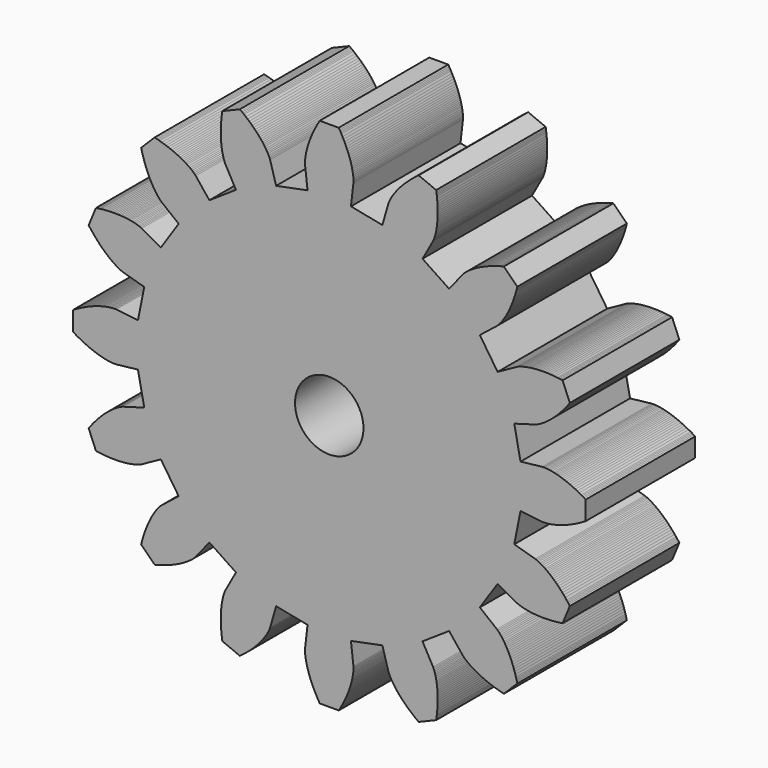
from build123d import *

# Parameters (mm, degrees)
F0_R     = 1.5
F1_DEPTH = 6


# Not quite as in the source:
# - ends of sketch curves that miss each other by under 0.0002 mm in the source are joined


with BuildPart() as f1:
    # F0 (on Front) → F1 (new body)
    with BuildSketch(Plane.XZ):
        with BuildLine():
            ThreePointArc((8.1098128622, -2.3285659726), (8.2466730878, -1.6403675501), (8.3835933696, -0.9521810736))
            Line((8.3835933696, -0.9521810736), (9.336897, -1.060451))
            Line((9.336897, -1.060451), (9.388357, -1.06268))
            Line((9.388357, -1.06268), (9.44023, -1.061917))
            Line((9.44023, -1.061917), (9.494537, -1.059018))
            Line((9.494537, -1.059018), (9.560114, -1.053224))
            Line((9.560114, -1.053224), (9.616606, -1.046504))
            Line((9.616606, -1.046504), (9.679275, -1.03738))
            Line((9.679275, -1.03738), (9.748033, -1.025526))
            Line((9.748033, -1.025526), (9.822771, -1.010618))
            Line((9.822771, -1.010618), (9.875862, -0.998824))
            Line((9.875862, -0.998824), (9.931523, -0.985435))
            Line((9.931523, -0.985435), (9.989713, -0.97036))
            Line((9.989713, -0.97036), (10.05039, -0.953506))
            Line((10.05039, -0.953506), (10.113507, -0.934781))
            Line((10.113507, -0.934781), (10.179017, -0.914096))
            Line((10.179017, -0.914096), (10.24687, -0.891361))
            Line((10.24687, -0.891361), (10.317014, -0.866489))
            Line((10.317014, -0.866489), (10.389394, -0.839394))
            Line((10.389394, -0.839394), (10.463954, -0.809989))
            Line((10.463954, -0.809989), (10.540633, -0.778191))
            Line((10.540633, -0.778191), (10.61937, -0.743918))
            Line((10.61937, -0.743918), (10.7001, -0.707087))
            Line((10.7001, -0.707087), (10.78276, -0.667621))
            Line((10.78276, -0.667621), (10.867278, -0.625439))
            Line((10.867278, -0.625439), (10.953587, -0.580466))
            Line((10.953587, -0.580466), (11.041613, -0.532627))
            Line((11.041613, -0.532627), (11.086246, -0.50761))
            Line((11.086246, -0.50761), (11.13128, -0.481849))
            Line((11.13128, -0.481849), (11.176706, -0.455335))
            Line((11.176706, -0.455335), (11.242303, -0.416041))
            Line((11.242303, -0.416041), (11.242301, 0.416042))
            Line((11.242301, 0.416042), (11.176705, 0.455336))
            Line((11.176705, 0.455336), (11.13128, 0.48185))
            Line((11.13128, 0.48185), (11.086245, 0.507611))
            Line((11.086245, 0.507611), (11.041612, 0.532628))
            Line((11.041612, 0.532628), (10.953587, 0.580467))
            Line((10.953587, 0.580467), (10.867277, 0.62544))
            Line((10.867277, 0.62544), (10.782758, 0.667622))
            Line((10.782758, 0.667622), (10.7001, 0.707089))
            Line((10.7001, 0.707089), (10.619369, 0.743919))
            Line((10.619369, 0.743919), (10.540632, 0.778193))
            Line((10.540632, 0.778193), (10.463953, 0.809991))
            Line((10.463953, 0.809991), (10.389394, 0.839395))
            Line((10.389394, 0.839395), (10.317014, 0.866491))
            Line((10.317014, 0.866491), (10.24687, 0.891362))
            Line((10.24687, 0.891362), (10.179016, 0.914097))
            Line((10.179016, 0.914097), (10.113507, 0.934782))
            Line((10.113507, 0.934782), (10.05039, 0.953507))
            Line((10.05039, 0.953507), (9.989712, 0.970362))
            Line((9.989712, 0.970362), (9.931522, 0.985437))
            Line((9.931522, 0.985437), (9.875862, 0.998825))
            Line((9.875862, 0.998825), (9.82277, 1.010619))
            Line((9.82277, 1.010619), (9.748032, 1.025527))
            Line((9.748032, 1.025527), (9.679275, 1.037381))
            Line((9.679275, 1.037381), (9.616605, 1.046505))
            Line((9.616605, 1.046505), (9.560113, 1.053226))
            Line((9.560113, 1.053226), (9.494536, 1.05902))
            Line((9.494536, 1.05902), (9.440229, 1.061919))
            Line((9.440229, 1.061919), (9.388357, 1.062681))
            Line((9.388357, 1.062681), (9.336897, 1.060452))
            Line((9.336897, 1.060452), (8.383598, 0.952181))
            ThreePointArc((8.383598, 0.952181), (8.2466779536, 1.640366924), (8.1098182701, 2.3285648549))
            Line((8.1098182701, 2.3285648549), (9.031984, 2.593346))
            Line((9.031984, 2.593346), (9.08038, 2.61098))
            Line((9.08038, 2.61098), (9.128012, 2.631536))
            Line((9.128012, 2.631536), (9.177077, 2.654996))
            Line((9.177077, 2.654996), (9.235444, 2.685445))
            Line((9.235444, 2.685445), (9.285064, 2.713272))
            Line((9.285064, 2.713272), (9.339471, 2.745684))
            Line((9.339471, 2.745684), (9.398459, 2.782947))
            Line((9.398459, 2.782947), (9.461803, 2.825322))
            Line((9.461803, 2.825322), (9.50634, 2.856535))
            Line((9.50634, 2.856535), (9.55264, 2.890205))
            Line((9.55264, 2.890205), (9.600631, 2.926401))
            Line((9.600631, 2.926401), (9.65024, 2.965193))
            Line((9.65024, 2.965193), (9.701386, 3.006646))
            Line((9.701386, 3.006646), (9.753994, 3.050826))
            Line((9.753994, 3.050826), (9.807982, 3.097797))
            Line((9.807982, 3.097797), (9.863268, 3.147618))
            Line((9.863268, 3.147618), (9.91977, 3.20035))
            Line((9.91977, 3.20035), (9.977402, 3.256049))
            Line((9.977402, 3.256049), (10.036075, 3.31477))
            Line((10.036075, 3.31477), (10.095703, 3.376566))
            Line((10.095703, 3.376566), (10.156193, 3.441487))
            Line((10.156193, 3.441487), (10.217458, 3.509582))
            Line((10.217458, 3.509582), (10.279401, 3.580897))
            Line((10.279401, 3.580897), (10.341929, 3.655475))
            Line((10.341929, 3.655475), (10.404946, 3.733358))
            Line((10.404946, 3.733358), (10.436609, 3.773552))
            Line((10.436609, 3.773552), (10.468356, 3.814586))
            Line((10.468356, 3.814586), (10.500178, 3.856465))
            Line((10.500178, 3.856465), (10.545745, 3.91787))
            Line((10.545745, 3.91787), (10.227319, 4.686615))
            Line((10.227319, 4.686615), (10.151679, 4.697815))
            Line((10.151679, 4.697815), (10.099564, 4.704927))
            Line((10.099564, 4.704927), (10.0481, 4.711493))
            Line((10.0481, 4.711493), (9.997291, 4.717525))
            Line((9.997291, 4.717525), (9.897658, 4.728037))
            Line((9.897658, 4.728037), (9.800709, 4.736558))
            Line((9.800709, 4.736558), (9.706481, 4.743185))
            Line((9.706481, 4.743185), (9.615012, 4.748015))
            Line((9.615012, 4.748015), (9.526332, 4.751148))
            Line((9.526332, 4.751148), (9.440472, 4.752681))
            Line((9.440472, 4.752681), (9.357462, 4.752715))
            Line((9.357462, 4.752715), (9.277326, 4.751348))
            Line((9.277326, 4.751348), (9.200086, 4.748683))
            Line((9.200086, 4.748683), (9.125763, 4.744818))
            Line((9.125763, 4.744818), (9.054374, 4.739856))
            Line((9.054374, 4.739856), (8.985936, 4.733897))
            Line((8.985936, 4.733897), (8.920458, 4.727043))
            Line((8.920458, 4.727043), (8.857949, 4.719394))
            Line((8.857949, 4.719394), (8.798419, 4.711053))
            Line((8.798419, 4.711053), (8.741873, 4.702122))
            Line((8.741873, 4.702122), (8.688308, 4.692701))
            Line((8.688308, 4.692701), (8.613554, 4.677873))
            Line((8.613554, 4.677873), (8.545495, 4.662513))
            Line((8.545495, 4.662513), (8.484104, 4.646959))
            Line((8.484104, 4.646959), (8.42934, 4.63155))
            Line((8.42934, 4.63155), (8.366538, 4.611807))
            Line((8.366538, 4.611807), (8.315254, 4.593703))
            Line((8.315254, 4.593703), (8.26704, 4.574557))
            Line((8.26704, 4.574557), (8.22035, 4.552805))
            Line((8.22035, 4.552805), (7.38105, 4.087963))
            ThreePointArc((7.38105, 4.087963), (6.9911949356, 4.6713679184), (6.6013908032, 5.2548068685))
            Line((6.6013908032, 5.2548068685), (7.352035, 5.852329))
            Line((7.352035, 5.852329), (7.389998, 5.887142))
            Line((7.389998, 5.887142), (7.426139, 5.92436))
            Line((7.426139, 5.92436), (7.46249, 5.964811))
            Line((7.46249, 5.964811), (7.504763, 6.015278))
            Line((7.504763, 6.015278), (7.539957, 6.059976))
            Line((7.539957, 6.059976), (7.577818, 6.110741))
            Line((7.577818, 6.110741), (7.618056, 6.167742))
            Line((7.618056, 6.167742), (7.660361, 6.231132))
            Line((7.660361, 6.231132), (7.689563, 6.277012))
            Line((7.689563, 6.277012), (7.719454, 6.325838))
            Line((7.719454, 6.325838), (7.749941, 6.377644))
            Line((7.749941, 6.377644), (7.780928, 6.432466))
            Line((7.780928, 6.432466), (7.812318, 6.490337))
            Line((7.812318, 6.490337), (7.844014, 6.551287))
            Line((7.844014, 6.551287), (7.875918, 6.615342))
            Line((7.875918, 6.615342), (7.907931, 6.682528))
            Line((7.907931, 6.682528), (7.939951, 6.752868))
            Line((7.939951, 6.752868), (7.971881, 6.826382))
            Line((7.971881, 6.826382), (8.003616, 6.903087))
            Line((8.003616, 6.903087), (8.035057, 6.982997))
            Line((8.035057, 6.982997), (8.066099, 7.066125))
            Line((8.066099, 7.066125), (8.096641, 7.152482))
            Line((8.096641, 7.152482), (8.126577, 7.242073))
            Line((8.126577, 7.242073), (8.155806, 7.334903))
            Line((8.155806, 7.334903), (8.184222, 7.430973))
            Line((8.184222, 7.430973), (8.198093, 7.480224))
            Line((8.198093, 7.480224), (8.211721, 7.530283))
            Line((8.211721, 7.530283), (8.225094, 7.581152))
            Line((8.225094, 7.581152), (8.243693, 7.65532))
            Line((8.243693, 7.65532), (7.65532, 8.243692))
            Line((7.65532, 8.243692), (7.581153, 8.225093))
            Line((7.581153, 8.225093), (7.530283, 8.211721))
            Line((7.530283, 8.211721), (7.480223, 8.198092))
            Line((7.480223, 8.198092), (7.430973, 8.184222))
            Line((7.430973, 8.184222), (7.334902, 8.155806))
            Line((7.334902, 8.155806), (7.242072, 8.126577))
            Line((7.242072, 8.126577), (7.152481, 8.096639))
            Line((7.152481, 8.096639), (7.066126, 8.066099))
            Line((7.066126, 8.066099), (6.982996, 8.035057))
            Line((6.982996, 8.035057), (6.903087, 8.003616))
            Line((6.903087, 8.003616), (6.826382, 7.97188))
            Line((6.826382, 7.97188), (6.752868, 7.939951))
            Line((6.752868, 7.939951), (6.682529, 7.90793))
            Line((6.682529, 7.90793), (6.615342, 7.875918))
            Line((6.615342, 7.875918), (6.551286, 7.844014))
            Line((6.551286, 7.844014), (6.490338, 7.812318))
            Line((6.490338, 7.812318), (6.432467, 7.780927))
            Line((6.432467, 7.780927), (6.377643, 7.749941))
            Line((6.377643, 7.749941), (6.325837, 7.719454))
            Line((6.325837, 7.719454), (6.277012, 7.689563))
            Line((6.277012, 7.689563), (6.231131, 7.660361))
            Line((6.231131, 7.660361), (6.167742, 7.618055))
            Line((6.167742, 7.618055), (6.110741, 7.577819))
            Line((6.110741, 7.577819), (6.059976, 7.539955))
            Line((6.059976, 7.539955), (6.015278, 7.504762))
            Line((6.015278, 7.504762), (5.96481, 7.462488))
            Line((5.96481, 7.462488), (5.92436, 7.426137))
            Line((5.92436, 7.426137), (5.887141, 7.389998))
            Line((5.887141, 7.389998), (5.85233, 7.352035))
            Line((5.85233, 7.352035), (5.254806, 6.601391))
            ThreePointArc((5.254806, 6.601391), (4.6713678902, 6.9911948934), (4.0879640006, 7.3810500008))
            Line((4.0879640006, 7.3810500008), (4.552805, 8.220348))
            Line((4.552805, 8.220348), (4.574556, 8.267039))
            Line((4.574556, 8.267039), (4.593703, 8.315255))
            Line((4.593703, 8.315255), (4.611807, 8.366537))
            Line((4.611807, 8.366537), (4.631549, 8.429341))
            Line((4.631549, 8.429341), (4.646959, 8.484103))
            Line((4.646959, 8.484103), (4.662513, 8.545494))
            Line((4.662513, 8.545494), (4.677873, 8.613554))
            Line((4.677873, 8.613554), (4.6927, 8.688308))
            Line((4.6927, 8.688308), (4.702121, 8.741871))
            Line((4.702121, 8.741871), (4.711053, 8.798419))
            Line((4.711053, 8.798419), (4.719393, 8.857949))
            Line((4.719393, 8.857949), (4.727042, 8.920456))
            Line((4.727042, 8.920456), (4.733896, 8.985934))
            Line((4.733896, 8.985934), (4.739855, 9.054374))
            Line((4.739855, 9.054374), (4.744818, 9.125763))
            Line((4.744818, 9.125763), (4.748682, 9.200085))
            Line((4.748682, 9.200085), (4.751347, 9.277325))
            Line((4.751347, 9.277325), (4.752714, 9.357462))
            Line((4.752714, 9.357462), (4.75268, 9.440471))
            Line((4.75268, 9.440471), (4.751147, 9.526331))
            Line((4.751147, 9.526331), (4.748014, 9.61501))
            Line((4.748014, 9.61501), (4.743184, 9.706481))
            Line((4.743184, 9.706481), (4.736557, 9.800708))
            Line((4.736557, 9.800708), (4.728037, 9.897657))
            Line((4.728037, 9.897657), (4.717525, 9.99729))
            Line((4.717525, 9.99729), (4.711492, 10.048099))
            Line((4.711492, 10.048099), (4.704926, 10.099564))
            Line((4.704926, 10.099564), (4.697815, 10.151679))
            Line((4.697815, 10.151679), (4.686615, 10.227319))
            Line((4.686615, 10.227319), (3.917869, 10.545742))
            Line((3.917869, 10.545742), (3.856464, 10.500177))
            Line((3.856464, 10.500177), (3.814585, 10.468356))
            Line((3.814585, 10.468356), (3.773551, 10.436607))
            Line((3.773551, 10.436607), (3.733358, 10.404945))
            Line((3.733358, 10.404945), (3.655474, 10.341927))
            Line((3.655474, 10.341927), (3.580896, 10.279398))
            Line((3.580896, 10.279398), (3.509581, 10.217455))
            Line((3.509581, 10.217455), (3.441486, 10.156192))
            Line((3.441486, 10.156192), (3.376565, 10.095701))
            Line((3.376565, 10.095701), (3.314769, 10.036073))
            Line((3.314769, 10.036073), (3.256047, 9.9774))
            Line((3.256047, 9.9774), (3.200349, 9.919769))
            Line((3.200349, 9.919769), (3.147617, 9.863268))
            Line((3.147617, 9.863268), (3.097796, 9.807982))
            Line((3.097796, 9.807982), (3.050826, 9.753992))
            Line((3.050826, 9.753992), (3.006645, 9.701385))
            Line((3.006645, 9.701385), (2.965192, 9.650238))
            Line((2.965192, 9.650238), (2.9264, 9.60063))
            Line((2.9264, 9.60063), (2.890204, 9.552638))
            Line((2.890204, 9.552638), (2.856535, 9.506338))
            Line((2.856535, 9.506338), (2.825321, 9.461801))
            Line((2.825321, 9.461801), (2.782947, 9.398458))
            Line((2.782947, 9.398458), (2.745683, 9.339471))
            Line((2.745683, 9.339471), (2.713271, 9.285062))
            Line((2.713271, 9.285062), (2.685444, 9.235443))
            Line((2.685444, 9.235443), (2.654995, 9.177075))
            Line((2.654995, 9.177075), (2.631534, 9.128011))
            Line((2.631534, 9.128011), (2.61098, 9.080379))
            Line((2.61098, 9.080379), (2.593345, 9.031984))
            Line((2.593345, 9.031984), (2.328564, 8.109817))
            ThreePointArc((2.328564, 8.109817), (1.6403660669, 8.2466771725), (0.9521800641, 8.3835973224))
            Line((0.9521800641, 8.3835973224), (1.060452, 9.336894))
            Line((1.060452, 9.336894), (1.06268, 9.388354))
            Line((1.06268, 9.388354), (1.061918, 9.440227))
            Line((1.061918, 9.440227), (1.059019, 9.494534))
            Line((1.059019, 9.494534), (1.053225, 9.560111))
            Line((1.053225, 9.560111), (1.046504, 9.616603))
            Line((1.046504, 9.616603), (1.03738, 9.679273))
            Line((1.03738, 9.679273), (1.025527, 9.74803))
            Line((1.025527, 9.74803), (1.010618, 9.822768))
            Line((1.010618, 9.822768), (0.998824, 9.875859))
            Line((0.998824, 9.875859), (0.985436, 9.931521))
            Line((0.985436, 9.931521), (0.970361, 9.98971))
            Line((0.970361, 9.98971), (0.953506, 10.050387))
            Line((0.953506, 10.050387), (0.934781, 10.113504))
            Line((0.934781, 10.113504), (0.914096, 10.179013))
            Line((0.914096, 10.179013), (0.891362, 10.246867))
            Line((0.891362, 10.246867), (0.86649, 10.317011))
            Line((0.86649, 10.317011), (0.839394, 10.389391))
            Line((0.839394, 10.389391), (0.80999, 10.463951))
            Line((0.80999, 10.463951), (0.778192, 10.540629))
            Line((0.778192, 10.540629), (0.743918, 10.619366))
            Line((0.743918, 10.619366), (0.707088, 10.700097))
            Line((0.707088, 10.700097), (0.667621, 10.782756))
            Line((0.667621, 10.782756), (0.62544, 10.867275))
            Line((0.62544, 10.867275), (0.580467, 10.953583))
            Line((0.580467, 10.953583), (0.532628, 11.041609))
            Line((0.532628, 11.041609), (0.50761, 11.086242))
            Line((0.50761, 11.086242), (0.481849, 11.131276))
            Line((0.481849, 11.131276), (0.455335, 11.176703))
            Line((0.455335, 11.176703), (0.416042, 11.242299))
            Line((0.416042, 11.242299), (-0.416042, 11.242299))
            Line((-0.416042, 11.242299), (-0.455335, 11.176703))
            Line((-0.455335, 11.176703), (-0.481849, 11.131277))
            Line((-0.481849, 11.131277), (-0.50761, 11.086242))
            Line((-0.50761, 11.086242), (-0.532628, 11.041609))
            Line((-0.532628, 11.041609), (-0.580466, 10.953584))
            Line((-0.580466, 10.953584), (-0.62544, 10.867275))
            Line((-0.62544, 10.867275), (-0.667621, 10.782756))
            Line((-0.667621, 10.782756), (-0.707088, 10.700097))
            Line((-0.707088, 10.700097), (-0.743918, 10.619366))
            Line((-0.743918, 10.619366), (-0.778192, 10.540629))
            Line((-0.778192, 10.540629), (-0.80999, 10.46395))
            Line((-0.80999, 10.46395), (-0.839395, 10.389392))
            Line((-0.839395, 10.389392), (-0.86649, 10.317011))
            Line((-0.86649, 10.317011), (-0.891362, 10.246868))
            Line((-0.891362, 10.246868), (-0.914096, 10.179013))
            Line((-0.914096, 10.179013), (-0.934781, 10.113504))
            Line((-0.934781, 10.113504), (-0.953506, 10.050388))
            Line((-0.953506, 10.050388), (-0.970361, 9.98971))
            Line((-0.970361, 9.98971), (-0.985436, 9.93152))
            Line((-0.985436, 9.93152), (-0.998824, 9.87586))
            Line((-0.998824, 9.87586), (-1.010618, 9.822768))
            Line((-1.010618, 9.822768), (-1.025527, 9.74803))
            Line((-1.025527, 9.74803), (-1.037381, 9.679273))
            Line((-1.037381, 9.679273), (-1.046504, 9.616603))
            Line((-1.046504, 9.616603), (-1.053225, 9.560111))
            Line((-1.053225, 9.560111), (-1.059019, 9.494534))
            Line((-1.059019, 9.494534), (-1.061918, 9.440227))
            Line((-1.061918, 9.440227), (-1.06268, 9.388355))
            Line((-1.06268, 9.388355), (-1.060452, 9.336895))
            Line((-1.060452, 9.336895), (-0.95218, 8.383596))
            ThreePointArc((-0.95218, 8.383596), (-1.6403666784, 8.2466772329), (-2.3285650902, 8.1098174538))
            Line((-2.3285650902, 8.1098174538), (-2.593346, 9.031983))
            Line((-2.593346, 9.031983), (-2.61098, 9.080378))
            Line((-2.61098, 9.080378), (-2.631535, 9.128011))
            Line((-2.631535, 9.128011), (-2.654996, 9.177075))
            Line((-2.654996, 9.177075), (-2.685444, 9.235442))
            Line((-2.685444, 9.235442), (-2.713272, 9.285061))
            Line((-2.713272, 9.285061), (-2.745683, 9.33947))
            Line((-2.745683, 9.33947), (-2.782947, 9.398457))
            Line((-2.782947, 9.398457), (-2.825322, 9.461801))
            Line((-2.825322, 9.461801), (-2.856535, 9.506337))
            Line((-2.856535, 9.506337), (-2.890205, 9.552638))
            Line((-2.890205, 9.552638), (-2.926401, 9.600629))
            Line((-2.926401, 9.600629), (-2.965192, 9.650237))
            Line((-2.965192, 9.650237), (-3.006645, 9.701384))
            Line((-3.006645, 9.701384), (-3.050826, 9.753992))
            Line((-3.050826, 9.753992), (-3.097796, 9.80798))
            Line((-3.097796, 9.80798), (-3.147618, 9.863266))
            Line((-3.147618, 9.863266), (-3.20035, 9.919768))
            Line((-3.20035, 9.919768), (-3.256049, 9.9774))
            Line((-3.256049, 9.9774), (-3.314769, 10.036073))
            Line((-3.314769, 10.036073), (-3.376566, 10.0957))
            Line((-3.376566, 10.0957), (-3.441487, 10.156191))
            Line((-3.441487, 10.156191), (-3.509582, 10.217456))
            Line((-3.509582, 10.217456), (-3.580896, 10.279398))
            Line((-3.580896, 10.279398), (-3.655475, 10.341926))
            Line((-3.655475, 10.341926), (-3.733358, 10.404944))
            Line((-3.733358, 10.404944), (-3.773552, 10.436606))
            Line((-3.773552, 10.436606), (-3.814586, 10.468354))
            Line((-3.814586, 10.468354), (-3.856465, 10.500176))
            Line((-3.856465, 10.500176), (-3.91787, 10.545743))
            Line((-3.91787, 10.545743), (-4.686615, 10.227317))
            Line((-4.686615, 10.227317), (-4.697815, 10.151677))
            Line((-4.697815, 10.151677), (-4.704926, 10.099563))
            Line((-4.704926, 10.099563), (-4.711492, 10.048098))
            Line((-4.711492, 10.048098), (-4.717525, 9.997289))
            Line((-4.717525, 9.997289), (-4.728037, 9.897656))
            Line((-4.728037, 9.897656), (-4.736557, 9.800707))
            Line((-4.736557, 9.800707), (-4.743185, 9.706479))
            Line((-4.743185, 9.706479), (-4.748015, 9.61501))
            Line((-4.748015, 9.61501), (-4.751147, 9.526329))
            Line((-4.751147, 9.526329), (-4.75268, 9.44047))
            Line((-4.75268, 9.44047), (-4.752715, 9.357459))
            Line((-4.752715, 9.357459), (-4.751348, 9.277324))
            Line((-4.751348, 9.277324), (-4.748682, 9.200084))
            Line((-4.748682, 9.200084), (-4.744818, 9.125762))
            Line((-4.744818, 9.125762), (-4.739855, 9.054372))
            Line((-4.739855, 9.054372), (-4.733896, 8.985934))
            Line((-4.733896, 8.985934), (-4.727042, 8.920456))
            Line((-4.727042, 8.920456), (-4.719393, 8.857947))
            Line((-4.719393, 8.857947), (-4.711053, 8.798417))
            Line((-4.711053, 8.798417), (-4.702122, 8.741871))
            Line((-4.702122, 8.741871), (-4.6927, 8.688307))
            Line((-4.6927, 8.688307), (-4.677873, 8.613552))
            Line((-4.677873, 8.613552), (-4.662513, 8.545494))
            Line((-4.662513, 8.545494), (-4.646959, 8.484103))
            Line((-4.646959, 8.484103), (-4.631549, 8.429338))
            Line((-4.631549, 8.429338), (-4.611807, 8.366536))
            Line((-4.611807, 8.366536), (-4.593703, 8.315254))
            Line((-4.593703, 8.315254), (-4.574556, 8.267038))
            Line((-4.574556, 8.267038), (-4.552805, 8.220348))
            Line((-4.552805, 8.220348), (-4.087963, 7.38105))
            ThreePointArc((-4.087963, 7.38105), (-4.671367156, 6.9911945428), (-5.254805702, 6.6013905539))
            Line((-5.254805702, 6.6013905539), (-5.85233, 7.352033))
            Line((-5.85233, 7.352033), (-5.887142, 7.389997))
            Line((-5.887142, 7.389997), (-5.924361, 7.426137))
            Line((-5.924361, 7.426137), (-5.964812, 7.462489))
            Line((-5.964812, 7.462489), (-6.015279, 7.504761))
            Line((-6.015279, 7.504761), (-6.059977, 7.539955))
            Line((-6.059977, 7.539955), (-6.110742, 7.577818))
            Line((-6.110742, 7.577818), (-6.167742, 7.618054))
            Line((-6.167742, 7.618054), (-6.231132, 7.66036))
            Line((-6.231132, 7.66036), (-6.277013, 7.689562))
            Line((-6.277013, 7.689562), (-6.325838, 7.719454))
            Line((-6.325838, 7.719454), (-6.377645, 7.749941))
            Line((-6.377645, 7.749941), (-6.432468, 7.780927))
            Line((-6.432468, 7.780927), (-6.490339, 7.812317))
            Line((-6.490339, 7.812317), (-6.551288, 7.844013))
            Line((-6.551288, 7.844013), (-6.615343, 7.875917))
            Line((-6.615343, 7.875917), (-6.68253, 7.907929))
            Line((-6.68253, 7.907929), (-6.75287, 7.939951))
            Line((-6.75287, 7.939951), (-6.826384, 7.971881))
            Line((-6.826384, 7.971881), (-6.903087, 8.003616))
            Line((-6.903087, 8.003616), (-6.982998, 8.035056))
            Line((-6.982998, 8.035056), (-7.066126, 8.066097))
            Line((-7.066126, 8.066097), (-7.152483, 8.09664))
            Line((-7.152483, 8.09664), (-7.242073, 8.126576))
            Line((-7.242073, 8.126576), (-7.334904, 8.155805))
            Line((-7.334904, 8.155805), (-7.430974, 8.184222))
            Line((-7.430974, 8.184222), (-7.480225, 8.198092))
            Line((-7.480225, 8.198092), (-7.530285, 8.21172))
            Line((-7.530285, 8.21172), (-7.581154, 8.225093))
            Line((-7.581154, 8.225093), (-7.655322, 8.243692))
            Line((-7.655322, 8.243692), (-8.243693, 7.655319))
            Line((-8.243693, 7.655319), (-8.225094, 7.581152))
            Line((-8.225094, 7.581152), (-8.211722, 7.530283))
            Line((-8.211722, 7.530283), (-8.198093, 7.480222))
            Line((-8.198093, 7.480222), (-8.184224, 7.430972))
            Line((-8.184224, 7.430972), (-8.155807, 7.334902))
            Line((-8.155807, 7.334902), (-8.126578, 7.242071))
            Line((-8.126578, 7.242071), (-8.09664, 7.15248))
            Line((-8.09664, 7.15248), (-8.0661, 7.066124))
            Line((-8.0661, 7.066124), (-8.035057, 6.982996))
            Line((-8.035057, 6.982996), (-8.003617, 6.903085))
            Line((-8.003617, 6.903085), (-7.971881, 6.826381))
            Line((-7.971881, 6.826381), (-7.939953, 6.752868))
            Line((-7.939953, 6.752868), (-7.907932, 6.682527))
            Line((-7.907932, 6.682527), (-7.875919, 6.615342))
            Line((-7.875919, 6.615342), (-7.844015, 6.551286))
            Line((-7.844015, 6.551286), (-7.812319, 6.490337))
            Line((-7.812319, 6.490337), (-7.780929, 6.432466))
            Line((-7.780929, 6.432466), (-7.749943, 6.377643))
            Line((-7.749943, 6.377643), (-7.719455, 6.325837))
            Line((-7.719455, 6.325837), (-7.689564, 6.277012))
            Line((-7.689564, 6.277012), (-7.660362, 6.23113))
            Line((-7.660362, 6.23113), (-7.618056, 6.167741))
            Line((-7.618056, 6.167741), (-7.57782, 6.110741))
            Line((-7.57782, 6.110741), (-7.539957, 6.059975))
            Line((-7.539957, 6.059975), (-7.504763, 6.015277))
            Line((-7.504763, 6.015277), (-7.46249, 5.96481))
            Line((-7.46249, 5.96481), (-7.426139, 5.924359))
            Line((-7.426139, 5.924359), (-7.389998, 5.887141))
            Line((-7.389998, 5.887141), (-7.352036, 5.852329))
            Line((-7.352036, 5.852329), (-6.601392, 5.254806))
            ThreePointArc((-6.601392, 5.254806), (-6.9911965642, 4.6713675043), (-7.381052057, 4.0879630381))
            Line((-7.381052057, 4.0879630381), (-8.22035, 4.552805))
            Line((-8.22035, 4.552805), (-8.267042, 4.574556))
            Line((-8.267042, 4.574556), (-8.315257, 4.593703))
            Line((-8.315257, 4.593703), (-8.366539, 4.611808))
            Line((-8.366539, 4.611808), (-8.429343, 4.631549))
            Line((-8.429343, 4.631549), (-8.484105, 4.646959))
            Line((-8.484105, 4.646959), (-8.545496, 4.662512))
            Line((-8.545496, 4.662512), (-8.613556, 4.677873))
            Line((-8.613556, 4.677873), (-8.68831, 4.6927))
            Line((-8.68831, 4.6927), (-8.741873, 4.702121))
            Line((-8.741873, 4.702121), (-8.798422, 4.711053))
            Line((-8.798422, 4.711053), (-8.857951, 4.719394))
            Line((-8.857951, 4.719394), (-8.920458, 4.727042))
            Line((-8.920458, 4.727042), (-8.985937, 4.733896))
            Line((-8.985937, 4.733896), (-9.054376, 4.739855))
            Line((-9.054376, 4.739855), (-9.125765, 4.744818))
            Line((-9.125765, 4.744818), (-9.200087, 4.748682))
            Line((-9.200087, 4.748682), (-9.277327, 4.751348))
            Line((-9.277327, 4.751348), (-9.357464, 4.752714))
            Line((-9.357464, 4.752714), (-9.440474, 4.752681))
            Line((-9.440474, 4.752681), (-9.526333, 4.751147))
            Line((-9.526333, 4.751147), (-9.615013, 4.748015))
            Line((-9.615013, 4.748015), (-9.706484, 4.743184))
            Line((-9.706484, 4.743184), (-9.800711, 4.736557))
            Line((-9.800711, 4.736557), (-9.89766, 4.728037))
            Line((-9.89766, 4.728037), (-9.997293, 4.717525))
            Line((-9.997293, 4.717525), (-10.048102, 4.711493))
            Line((-10.048102, 4.711493), (-10.099566, 4.704926))
            Line((-10.099566, 4.704926), (-10.151681, 4.697814))
            Line((-10.151681, 4.697814), (-10.227321, 4.686615))
            Line((-10.227321, 4.686615), (-10.545745, 3.91787))
            Line((-10.545745, 3.91787), (-10.500179, 3.856465))
            Line((-10.500179, 3.856465), (-10.468358, 3.814585))
            Line((-10.468358, 3.814585), (-10.436609, 3.773551))
            Line((-10.436609, 3.773551), (-10.404947, 3.733358))
            Line((-10.404947, 3.733358), (-10.34193, 3.655475))
            Line((-10.34193, 3.655475), (-10.279401, 3.580896))
            Line((-10.279401, 3.580896), (-10.217458, 3.509581))
            Line((-10.217458, 3.509581), (-10.156195, 3.441487))
            Line((-10.156195, 3.441487), (-10.095703, 3.376565))
            Line((-10.095703, 3.376565), (-10.036076, 3.31477))
            Line((-10.036076, 3.31477), (-9.977402, 3.256048))
            Line((-9.977402, 3.256048), (-9.919771, 3.20035))
            Line((-9.919771, 3.20035), (-9.86327, 3.147618))
            Line((-9.86327, 3.147618), (-9.807984, 3.097797))
            Line((-9.807984, 3.097797), (-9.753994, 3.050826))
            Line((-9.753994, 3.050826), (-9.701387, 3.006646))
            Line((-9.701387, 3.006646), (-9.650241, 2.965193))
            Line((-9.650241, 2.965193), (-9.600632, 2.926401))
            Line((-9.600632, 2.926401), (-9.55264, 2.890205))
            Line((-9.55264, 2.890205), (-9.50634, 2.856536))
            Line((-9.50634, 2.856536), (-9.461804, 2.825322))
            Line((-9.461804, 2.825322), (-9.39846, 2.782947))
            Line((-9.39846, 2.782947), (-9.339473, 2.745684))
            Line((-9.339473, 2.745684), (-9.285064, 2.713272))
            Line((-9.285064, 2.713272), (-9.235445, 2.685445))
            Line((-9.235445, 2.685445), (-9.177077, 2.654996))
            Line((-9.177077, 2.654996), (-9.128013, 2.631535))
            Line((-9.128013, 2.631535), (-9.080382, 2.61098))
            Line((-9.080382, 2.61098), (-9.031986, 2.593346))
            Line((-9.031986, 2.593346), (-8.109819, 2.328565))
            ThreePointArc((-8.109819, 2.328565), (-8.2466793482, 1.6403671019), (-8.3835995704, 0.9521811135))
            Line((-8.3835995704, 0.9521811135), (-9.336897, 1.060453))
            Line((-9.336897, 1.060453), (-9.388357, 1.062681))
            Line((-9.388357, 1.062681), (-9.44023, 1.061919))
            Line((-9.44023, 1.061919), (-9.494537, 1.05902))
            Line((-9.494537, 1.05902), (-9.560114, 1.053226))
            Line((-9.560114, 1.053226), (-9.616606, 1.046505))
            Line((-9.616606, 1.046505), (-9.679275, 1.037381))
            Line((-9.679275, 1.037381), (-9.748033, 1.025528))
            Line((-9.748033, 1.025528), (-9.822771, 1.010619))
            Line((-9.822771, 1.010619), (-9.875862, 0.998825))
            Line((-9.875862, 0.998825), (-9.931523, 0.985437))
            Line((-9.931523, 0.985437), (-9.989713, 0.970362))
            Line((-9.989713, 0.970362), (-10.05039, 0.953507))
            Line((-10.05039, 0.953507), (-10.113507, 0.934782))
            Line((-10.113507, 0.934782), (-10.179017, 0.914097))
            Line((-10.179017, 0.914097), (-10.24687, 0.891363))
            Line((-10.24687, 0.891363), (-10.317014, 0.866491))
            Line((-10.317014, 0.866491), (-10.389394, 0.839395))
            Line((-10.389394, 0.839395), (-10.463954, 0.809991))
            Line((-10.463954, 0.809991), (-10.540633, 0.778193))
            Line((-10.540633, 0.778193), (-10.61937, 0.74392))
            Line((-10.61937, 0.74392), (-10.7001, 0.707089))
            Line((-10.7001, 0.707089), (-10.78276, 0.667622))
            Line((-10.78276, 0.667622), (-10.867278, 0.625441))
            Line((-10.867278, 0.625441), (-10.953587, 0.580468))
            Line((-10.953587, 0.580468), (-11.041613, 0.532629))
            Line((-11.041613, 0.532629), (-11.086246, 0.507611))
            Line((-11.086246, 0.507611), (-11.13128, 0.48185))
            Line((-11.13128, 0.48185), (-11.176706, 0.455336))
            Line((-11.176706, 0.455336), (-11.242303, 0.416043))
            Line((-11.242303, 0.416043), (-11.242301, -0.41604))
            Line((-11.242301, -0.41604), (-11.176705, -0.455334))
            Line((-11.176705, -0.455334), (-11.13128, -0.481848))
            Line((-11.13128, -0.481848), (-11.086245, -0.507609))
            Line((-11.086245, -0.507609), (-11.041612, -0.532626))
            Line((-11.041612, -0.532626), (-10.953587, -0.580465))
            Line((-10.953587, -0.580465), (-10.867277, -0.625438))
            Line((-10.867277, -0.625438), (-10.782758, -0.66762))
            Line((-10.782758, -0.66762), (-10.7001, -0.707087))
            Line((-10.7001, -0.707087), (-10.619369, -0.743917))
            Line((-10.619369, -0.743917), (-10.540632, -0.77819))
            Line((-10.540632, -0.77819), (-10.463953, -0.809988))
            Line((-10.463953, -0.809988), (-10.389394, -0.839393))
            Line((-10.389394, -0.839393), (-10.317014, -0.866488))
            Line((-10.317014, -0.866488), (-10.24687, -0.89136))
            Line((-10.24687, -0.89136), (-10.179016, -0.914095))
            Line((-10.179016, -0.914095), (-10.113507, -0.93478))
            Line((-10.113507, -0.93478), (-10.05039, -0.953505))
            Line((-10.05039, -0.953505), (-9.989712, -0.970359))
            Line((-9.989712, -0.970359), (-9.931522, -0.985434))
            Line((-9.931522, -0.985434), (-9.875862, -0.998823))
            Line((-9.875862, -0.998823), (-9.82277, -1.010617))
            Line((-9.82277, -1.010617), (-9.748032, -1.025525))
            Line((-9.748032, -1.025525), (-9.679275, -1.037379))
            Line((-9.679275, -1.037379), (-9.616605, -1.046502))
            Line((-9.616605, -1.046502), (-9.560113, -1.053223))
            Line((-9.560113, -1.053223), (-9.494536, -1.059017))
            Line((-9.494536, -1.059017), (-9.440229, -1.061916))
            Line((-9.440229, -1.061916), (-9.388357, -1.062678))
            Line((-9.388357, -1.062678), (-9.336897, -1.06045))
            Line((-9.336897, -1.06045), (-8.383598, -0.952178))
            ThreePointArc((-8.383598, -0.952178), (-8.2466786079, -1.6403645541), (-8.1098187744, -2.3285629551))
            Line((-8.1098187744, -2.3285629551), (-9.031986, -2.593344))
            Line((-9.031986, -2.593344), (-9.080382, -2.610978))
            Line((-9.080382, -2.610978), (-9.128014, -2.631533))
            Line((-9.128014, -2.631533), (-9.177078, -2.654993))
            Line((-9.177078, -2.654993), (-9.235446, -2.685442))
            Line((-9.235446, -2.685442), (-9.285066, -2.71327))
            Line((-9.285066, -2.71327), (-9.339474, -2.745681))
            Line((-9.339474, -2.745681), (-9.398461, -2.782945))
            Line((-9.398461, -2.782945), (-9.461804, -2.825319))
            Line((-9.461804, -2.825319), (-9.506342, -2.856533))
            Line((-9.506342, -2.856533), (-9.552642, -2.890203))
            Line((-9.552642, -2.890203), (-9.600634, -2.926399))
            Line((-9.600634, -2.926399), (-9.650242, -2.96519))
            Line((-9.650242, -2.96519), (-9.701388, -3.006643))
            Line((-9.701388, -3.006643), (-9.753996, -3.050823))
            Line((-9.753996, -3.050823), (-9.807984, -3.097794))
            Line((-9.807984, -3.097794), (-9.86327, -3.147615))
            Line((-9.86327, -3.147615), (-9.919772, -3.200347))
            Line((-9.919772, -3.200347), (-9.977404, -3.256046))
            Line((-9.977404, -3.256046), (-10.036077, -3.314767))
            Line((-10.036077, -3.314767), (-10.095705, -3.376563))
            Line((-10.095705, -3.376563), (-10.156196, -3.441484))
            Line((-10.156196, -3.441484), (-10.21746, -3.509579))
            Line((-10.21746, -3.509579), (-10.279403, -3.580894))
            Line((-10.279403, -3.580894), (-10.341931, -3.655472))
            Line((-10.341931, -3.655472), (-10.404949, -3.733356))
            Line((-10.404949, -3.733356), (-10.436611, -3.773549))
            Line((-10.436611, -3.773549), (-10.468359, -3.814583))
            Line((-10.468359, -3.814583), (-10.50018, -3.856462))
            Line((-10.50018, -3.856462), (-10.545748, -3.917868))
            Line((-10.545748, -3.917868), (-10.227321, -4.686612))
            Line((-10.227321, -4.686612), (-10.151681, -4.697812))
            Line((-10.151681, -4.697812), (-10.099567, -4.704924))
            Line((-10.099567, -4.704924), (-10.048102, -4.71149))
            Line((-10.048102, -4.71149), (-9.997293, -4.717522))
            Line((-9.997293, -4.717522), (-9.897661, -4.728034))
            Line((-9.897661, -4.728034), (-9.800711, -4.736555))
            Line((-9.800711, -4.736555), (-9.706483, -4.743181))
            Line((-9.706483, -4.743181), (-9.615014, -4.748012))
            Line((-9.615014, -4.748012), (-9.526334, -4.751145))
            Line((-9.526334, -4.751145), (-9.440474, -4.752678))
            Line((-9.440474, -4.752678), (-9.357463, -4.752712))
            Line((-9.357463, -4.752712), (-9.277328, -4.751346))
            Line((-9.277328, -4.751346), (-9.200088, -4.74868))
            Line((-9.200088, -4.74868), (-9.125765, -4.744816))
            Line((-9.125765, -4.744816), (-9.054376, -4.739853))
            Line((-9.054376, -4.739853), (-8.985938, -4.733894))
            Line((-8.985938, -4.733894), (-8.92046, -4.727039))
            Line((-8.92046, -4.727039), (-8.857951, -4.719391))
            Line((-8.857951, -4.719391), (-8.798421, -4.71105))
            Line((-8.798421, -4.71105), (-8.741875, -4.702119))
            Line((-8.741875, -4.702119), (-8.68831, -4.692698))
            Line((-8.68831, -4.692698), (-8.613556, -4.677871))
            Line((-8.613556, -4.677871), (-8.545497, -4.66251))
            Line((-8.545497, -4.66251), (-8.484106, -4.646956))
            Line((-8.484106, -4.646956), (-8.429343, -4.631547))
            Line((-8.429343, -4.631547), (-8.36654, -4.611805))
            Line((-8.36654, -4.611805), (-8.315257, -4.5937))
            Line((-8.315257, -4.5937), (-8.267042, -4.574554))
            Line((-8.267042, -4.574554), (-8.220352, -4.552802))
            Line((-8.220352, -4.552802), (-7.381052, -4.087961))
            ThreePointArc((-7.381052, -4.087961), (-6.9911976105, -4.6713653693), (-6.6013937652, -5.2548035112))
            Line((-6.6013937652, -5.2548035112), (-7.352037, -5.852327))
            Line((-7.352037, -5.852327), (-7.390001, -5.887139))
            Line((-7.390001, -5.887139), (-7.426142, -5.924358))
            Line((-7.426142, -5.924358), (-7.462493, -5.964808))
            Line((-7.462493, -5.964808), (-7.504766, -6.015276))
            Line((-7.504766, -6.015276), (-7.53996, -6.059973))
            Line((-7.53996, -6.059973), (-7.577821, -6.110739))
            Line((-7.577821, -6.110739), (-7.618059, -6.167739))
            Line((-7.618059, -6.167739), (-7.660365, -6.231129))
            Line((-7.660365, -6.231129), (-7.689566, -6.27701))
            Line((-7.689566, -6.27701), (-7.719458, -6.325835))
            Line((-7.719458, -6.325835), (-7.749945, -6.377642))
            Line((-7.749945, -6.377642), (-7.780932, -6.432464))
            Line((-7.780932, -6.432464), (-7.812321, -6.490335))
            Line((-7.812321, -6.490335), (-7.844018, -6.551285))
            Line((-7.844018, -6.551285), (-7.875922, -6.61534))
            Line((-7.875922, -6.61534), (-7.907934, -6.682525))
            Line((-7.907934, -6.682525), (-7.939955, -6.752866))
            Line((-7.939955, -6.752866), (-7.971885, -6.82638))
            Line((-7.971885, -6.82638), (-8.00362, -6.903084))
            Line((-8.00362, -6.903084), (-8.035061, -6.982995))
            Line((-8.035061, -6.982995), (-8.066102, -7.066122))
            Line((-8.066102, -7.066122), (-8.096644, -7.152479))
            Line((-8.096644, -7.152479), (-8.12658, -7.24207))
            Line((-8.12658, -7.24207), (-8.155809, -7.3349))
            Line((-8.155809, -7.3349), (-8.184226, -7.430971))
            Line((-8.184226, -7.430971), (-8.198096, -7.480221))
            Line((-8.198096, -7.480221), (-8.211724, -7.530281))
            Line((-8.211724, -7.530281), (-8.225098, -7.58115))
            Line((-8.225098, -7.58115), (-8.243697, -7.655319))
            Line((-8.243697, -7.655319), (-7.655324, -8.243689))
            Line((-7.655324, -8.243689), (-7.581156, -8.22509))
            Line((-7.581156, -8.22509), (-7.530287, -8.211718))
            Line((-7.530287, -8.211718), (-7.480227, -8.198089))
            Line((-7.480227, -8.198089), (-7.430977, -8.184219))
            Line((-7.430977, -8.184219), (-7.334905, -8.155803))
            Line((-7.334905, -8.155803), (-7.242075, -8.126574))
            Line((-7.242075, -8.126574), (-7.152485, -8.096637))
            Line((-7.152485, -8.096637), (-7.066129, -8.066096))
            Line((-7.066129, -8.066096), (-6.983, -8.035054))
            Line((-6.983, -8.035054), (-6.90309, -8.003613))
            Line((-6.90309, -8.003613), (-6.826385, -7.971877))
            Line((-6.826385, -7.971877), (-6.752872, -7.939949))
            Line((-6.752872, -7.939949), (-6.682532, -7.907928))
            Line((-6.682532, -7.907928), (-6.615346, -7.875916))
            Line((-6.615346, -7.875916), (-6.55129, -7.844011))
            Line((-6.55129, -7.844011), (-6.490341, -7.812316))
            Line((-6.490341, -7.812316), (-6.432471, -7.780925))
            Line((-6.432471, -7.780925), (-6.377647, -7.749938))
            Line((-6.377647, -7.749938), (-6.32584, -7.719451))
            Line((-6.32584, -7.719451), (-6.277015, -7.689561))
            Line((-6.277015, -7.689561), (-6.231134, -7.660359))
            Line((-6.231134, -7.660359), (-6.167744, -7.618053))
            Line((-6.167744, -7.618053), (-6.110744, -7.577817))
            Line((-6.110744, -7.577817), (-6.059978, -7.539953))
            Line((-6.059978, -7.539953), (-6.01528, -7.50476))
            Line((-6.01528, -7.50476), (-5.964813, -7.462486))
            Line((-5.964813, -7.462486), (-5.924362, -7.426135))
            Line((-5.924362, -7.426135), (-5.887145, -7.389996))
            Line((-5.887145, -7.389996), (-5.852332, -7.352033))
            Line((-5.852332, -7.352033), (-5.254808, -6.601389))
            ThreePointArc((-5.254808, -6.601389), (-4.6713698053, -6.9911935145), (-4.0879655116, -7.3810487656))
            Line((-4.0879655116, -7.3810487656), (-4.552807, -8.220347))
            Line((-4.552807, -8.220347), (-4.57456, -8.267038))
            Line((-4.57456, -8.267038), (-4.593706, -8.315253))
            Line((-4.593706, -8.315253), (-4.61181, -8.366536))
            Line((-4.61181, -8.366536), (-4.631552, -8.429339))
            Line((-4.631552, -8.429339), (-4.646962, -8.484101))
            Line((-4.646962, -8.484101), (-4.662515, -8.545493))
            Line((-4.662515, -8.545493), (-4.677876, -8.613552))
            Line((-4.677876, -8.613552), (-4.692704, -8.688306))
            Line((-4.692704, -8.688306), (-4.702124, -8.741869))
            Line((-4.702124, -8.741869), (-4.711056, -8.798418))
            Line((-4.711056, -8.798418), (-4.719397, -8.857947))
            Line((-4.719397, -8.857947), (-4.727045, -8.920454))
            Line((-4.727045, -8.920454), (-4.733899, -8.985933))
            Line((-4.733899, -8.985933), (-4.739858, -9.054372))
            Line((-4.739858, -9.054372), (-4.744821, -9.125761))
            Line((-4.744821, -9.125761), (-4.748685, -9.200083))
            Line((-4.748685, -9.200083), (-4.751351, -9.277323))
            Line((-4.751351, -9.277323), (-4.752718, -9.35746))
            Line((-4.752718, -9.35746), (-4.752683, -9.44047))
            Line((-4.752683, -9.44047), (-4.75115, -9.526329))
            Line((-4.75115, -9.526329), (-4.748017, -9.615009))
            Line((-4.748017, -9.615009), (-4.743188, -9.70648))
            Line((-4.743188, -9.70648), (-4.736561, -9.800707))
            Line((-4.736561, -9.800707), (-4.72804, -9.897655))
            Line((-4.72804, -9.897655), (-4.717529, -9.997289))
            Line((-4.717529, -9.997289), (-4.711496, -10.048097))
            Line((-4.711496, -10.048097), (-4.704929, -10.099562))
            Line((-4.704929, -10.099562), (-4.697818, -10.151677))
            Line((-4.697818, -10.151677), (-4.686618, -10.227317))
            Line((-4.686618, -10.227317), (-3.917873, -10.545741))
            Line((-3.917873, -10.545741), (-3.856468, -10.500175))
            Line((-3.856468, -10.500175), (-3.814589, -10.468354))
            Line((-3.814589, -10.468354), (-3.773554, -10.436605))
            Line((-3.773554, -10.436605), (-3.733361, -10.404943))
            Line((-3.733361, -10.404943), (-3.655478, -10.341925))
            Line((-3.655478, -10.341925), (-3.580899, -10.279397))
            Line((-3.580899, -10.279397), (-3.509584, -10.217454))
            Line((-3.509584, -10.217454), (-3.441489, -10.156191))
            Line((-3.441489, -10.156191), (-3.376568, -10.095699))
            Line((-3.376568, -10.095699), (-3.314772, -10.036072))
            Line((-3.314772, -10.036072), (-3.256051, -9.977398))
            Line((-3.256051, -9.977398), (-3.200352, -9.919767))
            Line((-3.200352, -9.919767), (-3.14762, -9.863266))
            Line((-3.14762, -9.863266), (-3.097799, -9.80798))
            Line((-3.097799, -9.80798), (-3.050828, -9.75399))
            Line((-3.050828, -9.75399), (-3.006649, -9.701383))
            Line((-3.006649, -9.701383), (-2.965195, -9.650237))
            Line((-2.965195, -9.650237), (-2.926403, -9.600628))
            Line((-2.926403, -9.600628), (-2.890207, -9.552636))
            Line((-2.890207, -9.552636), (-2.856538, -9.506336))
            Line((-2.856538, -9.506336), (-2.825324, -9.4618))
            Line((-2.825324, -9.4618), (-2.782949, -9.398455))
            Line((-2.782949, -9.398455), (-2.745686, -9.33947))
            Line((-2.745686, -9.33947), (-2.713274, -9.285061))
            Line((-2.713274, -9.285061), (-2.685446, -9.235441))
            Line((-2.685446, -9.235441), (-2.654998, -9.177073))
            Line((-2.654998, -9.177073), (-2.631537, -9.12801))
            Line((-2.631537, -9.12801), (-2.610983, -9.080378))
            Line((-2.610983, -9.080378), (-2.593348, -9.031982))
            Line((-2.593348, -9.031982), (-2.328567, -8.109815))
            ThreePointArc((-2.328567, -8.109815), (-1.6403685246, -8.2466754596), (-0.9521819451, -8.3835957242))
            Line((-0.9521819451, -8.3835957242), (-1.060455, -9.336894))
            Line((-1.060455, -9.336894), (-1.062683, -9.388354))
            Line((-1.062683, -9.388354), (-1.061921, -9.440226))
            Line((-1.061921, -9.440226), (-1.059022, -9.494534))
            Line((-1.059022, -9.494534), (-1.053228, -9.560111))
            Line((-1.053228, -9.560111), (-1.046507, -9.616603))
            Line((-1.046507, -9.616603), (-1.037383, -9.679272))
            Line((-1.037383, -9.679272), (-1.02553, -9.748029))
            Line((-1.02553, -9.748029), (-1.010621, -9.822767))
            Line((-1.010621, -9.822767), (-0.998827, -9.875859))
            Line((-0.998827, -9.875859), (-0.985439, -9.93152))
            Line((-0.985439, -9.93152), (-0.970364, -9.98971))
            Line((-0.970364, -9.98971), (-0.953509, -10.050386))
            Line((-0.953509, -10.050386), (-0.934785, -10.113503))
            Line((-0.934785, -10.113503), (-0.914099, -10.179013))
            Line((-0.914099, -10.179013), (-0.891365, -10.246866))
            Line((-0.891365, -10.246866), (-0.866493, -10.31701))
            Line((-0.866493, -10.31701), (-0.839398, -10.38939))
            Line((-0.839398, -10.38939), (-0.809993, -10.46395))
            Line((-0.809993, -10.46395), (-0.778195, -10.540629))
            Line((-0.778195, -10.540629), (-0.743922, -10.619366))
            Line((-0.743922, -10.619366), (-0.707091, -10.700096))
            Line((-0.707091, -10.700096), (-0.667624, -10.782756))
            Line((-0.667624, -10.782756), (-0.625443, -10.867274))
            Line((-0.625443, -10.867274), (-0.58047, -10.953583))
            Line((-0.58047, -10.953583), (-0.532631, -11.041609))
            Line((-0.532631, -11.041609), (-0.507614, -11.086242))
            Line((-0.507614, -11.086242), (-0.481853, -11.131276))
            Line((-0.481853, -11.131276), (-0.455339, -11.176702))
            Line((-0.455339, -11.176702), (-0.416045, -11.242299))
            Line((-0.416045, -11.242299), (0.416038, -11.242298))
            Line((0.416038, -11.242298), (0.455332, -11.176702))
            Line((0.455332, -11.176702), (0.481846, -11.131277))
            Line((0.481846, -11.131277), (0.507607, -11.086242))
            Line((0.507607, -11.086242), (0.532624, -11.041609))
            Line((0.532624, -11.041609), (0.580463, -10.953583))
            Line((0.580463, -10.953583), (0.625436, -10.867274))
            Line((0.625436, -10.867274), (0.667618, -10.782755))
            Line((0.667618, -10.782755), (0.707085, -10.700097))
            Line((0.707085, -10.700097), (0.743915, -10.619366))
            Line((0.743915, -10.619366), (0.778189, -10.540629))
            Line((0.778189, -10.540629), (0.809987, -10.46395))
            Line((0.809987, -10.46395), (0.839391, -10.389391))
            Line((0.839391, -10.389391), (0.866487, -10.317011))
            Line((0.866487, -10.317011), (0.891358, -10.246867))
            Line((0.891358, -10.246867), (0.914093, -10.179013))
            Line((0.914093, -10.179013), (0.934778, -10.113504))
            Line((0.934778, -10.113504), (0.953503, -10.050387))
            Line((0.953503, -10.050387), (0.970358, -9.98971))
            Line((0.970358, -9.98971), (0.985433, -9.931519))
            Line((0.985433, -9.931519), (0.998821, -9.87586))
            Line((0.998821, -9.87586), (1.010615, -9.822767))
            Line((1.010615, -9.822767), (1.025524, -9.748029))
            Line((1.025524, -9.748029), (1.037378, -9.679273))
            Line((1.037378, -9.679273), (1.046501, -9.616603))
            Line((1.046501, -9.616603), (1.053222, -9.560111))
            Line((1.053222, -9.560111), (1.059016, -9.494534))
            Line((1.059016, -9.494534), (1.061915, -9.440226))
            Line((1.061915, -9.440226), (1.062677, -9.388354))
            Line((1.062677, -9.388354), (1.060449, -9.336894))
            Line((1.060449, -9.336894), (0.952177, -8.383596))
            ThreePointArc((0.952177, -8.383596), (1.6403633813, -8.2466752392), (2.3285618817, -8.1098154048))
            Line((2.3285618817, -8.1098154048), (2.593342, -9.031983))
            Line((2.593342, -9.031983), (2.610976, -9.080378))
            Line((2.610976, -9.080378), (2.631531, -9.128011))
            Line((2.631531, -9.128011), (2.654992, -9.177075))
            Line((2.654992, -9.177075), (2.68544, -9.235443))
            Line((2.68544, -9.235443), (2.713268, -9.285062))
            Line((2.713268, -9.285062), (2.745679, -9.33947))
            Line((2.745679, -9.33947), (2.782943, -9.398458))
            Line((2.782943, -9.398458), (2.825317, -9.461801))
            Line((2.825317, -9.461801), (2.856531, -9.506338))
            Line((2.856531, -9.506338), (2.890201, -9.552639))
            Line((2.890201, -9.552639), (2.926397, -9.60063))
            Line((2.926397, -9.60063), (2.965188, -9.650237))
            Line((2.965188, -9.650237), (3.006641, -9.701384))
            Line((3.006641, -9.701384), (3.050822, -9.753993))
            Line((3.050822, -9.753993), (3.097792, -9.807981))
            Line((3.097792, -9.807981), (3.147613, -9.863267))
            Line((3.147613, -9.863267), (3.200345, -9.919769))
            Line((3.200345, -9.919769), (3.256044, -9.977401))
            Line((3.256044, -9.977401), (3.314765, -10.036073))
            Line((3.314765, -10.036073), (3.376561, -10.095701))
            Line((3.376561, -10.095701), (3.441482, -10.156192))
            Line((3.441482, -10.156192), (3.509577, -10.217456))
            Line((3.509577, -10.217456), (3.580892, -10.279398))
            Line((3.580892, -10.279398), (3.65547, -10.341927))
            Line((3.65547, -10.341927), (3.733353, -10.404945))
            Line((3.733353, -10.404945), (3.773547, -10.436607))
            Line((3.773547, -10.436607), (3.814581, -10.468355))
            Line((3.814581, -10.468355), (3.85646, -10.500177))
            Line((3.85646, -10.500177), (3.917865, -10.545744))
            Line((3.917865, -10.545744), (4.68661, -10.227317))
            Line((4.68661, -10.227317), (4.69781, -10.151678))
            Line((4.69781, -10.151678), (4.704922, -10.099564))
            Line((4.704922, -10.099564), (4.711488, -10.048098))
            Line((4.711488, -10.048098), (4.717521, -9.99729))
            Line((4.717521, -9.99729), (4.728032, -9.897657))
            Line((4.728032, -9.897657), (4.736553, -9.800707))
            Line((4.736553, -9.800707), (4.74318, -9.706479))
            Line((4.74318, -9.706479), (4.74801, -9.61501))
            Line((4.74801, -9.61501), (4.751143, -9.526331))
            Line((4.751143, -9.526331), (4.752676, -9.44047))
            Line((4.752676, -9.44047), (4.75271, -9.35746))
            Line((4.75271, -9.35746), (4.751344, -9.277325))
            Line((4.751344, -9.277325), (4.748678, -9.200085))
            Line((4.748678, -9.200085), (4.744814, -9.125763))
            Line((4.744814, -9.125763), (4.739851, -9.054373))
            Line((4.739851, -9.054373), (4.733892, -8.985934))
            Line((4.733892, -8.985934), (4.727038, -8.920456))
            Line((4.727038, -8.920456), (4.719389, -8.857948))
            Line((4.719389, -8.857948), (4.711049, -8.798418))
            Line((4.711049, -8.798418), (4.702117, -8.741872))
            Line((4.702117, -8.741872), (4.692696, -8.688307))
            Line((4.692696, -8.688307), (4.677869, -8.613553))
            Line((4.677869, -8.613553), (4.662508, -8.545494))
            Line((4.662508, -8.545494), (4.646955, -8.484103))
            Line((4.646955, -8.484103), (4.631545, -8.429339))
            Line((4.631545, -8.429339), (4.611803, -8.366537))
            Line((4.611803, -8.366537), (4.593699, -8.315254))
            Line((4.593699, -8.315254), (4.574553, -8.267038))
            Line((4.574553, -8.267038), (4.552801, -8.220349))
            Line((4.552801, -8.220349), (4.087959, -7.38105))
            ThreePointArc((4.087959, -7.38105), (4.6713633751, -6.9911948708), (5.2548019211, -6.6013908819))
            Line((5.2548019211, -6.6013908819), (5.852325, -7.352035))
            Line((5.852325, -7.352035), (5.887137, -7.389998))
            Line((5.887137, -7.389998), (5.924355, -7.426139))
            Line((5.924355, -7.426139), (5.964807, -7.46249))
            Line((5.964807, -7.46249), (6.015273, -7.504763))
            Line((6.015273, -7.504763), (6.059971, -7.539956))
            Line((6.059971, -7.539956), (6.110737, -7.577819))
            Line((6.110737, -7.577819), (6.167737, -7.618055))
            Line((6.167737, -7.618055), (6.231127, -7.660361))
            Line((6.231127, -7.660361), (6.277008, -7.689563))
            Line((6.277008, -7.689563), (6.325833, -7.719455))
            Line((6.325833, -7.719455), (6.37764, -7.749942))
            Line((6.37764, -7.749942), (6.432462, -7.780928))
            Line((6.432462, -7.780928), (6.490333, -7.812319))
            Line((6.490333, -7.812319), (6.551283, -7.844014))
            Line((6.551283, -7.844014), (6.615337, -7.875918))
            Line((6.615337, -7.875918), (6.682523, -7.907931))
            Line((6.682523, -7.907931), (6.752863, -7.939952))
            Line((6.752863, -7.939952), (6.826377, -7.971882))
            Line((6.826377, -7.971882), (6.903082, -8.003617))
            Line((6.903082, -8.003617), (6.982992, -8.035057))
            Line((6.982992, -8.035057), (7.06612, -8.066099))
            Line((7.06612, -8.066099), (7.152477, -8.096642))
            Line((7.152477, -8.096642), (7.242067, -8.126577))
            Line((7.242067, -8.126577), (7.334898, -8.155806))
            Line((7.334898, -8.155806), (7.430968, -8.184223))
            Line((7.430968, -8.184223), (7.480219, -8.198094))
            Line((7.480219, -8.198094), (7.530279, -8.211721))
            Line((7.530279, -8.211721), (7.581148, -8.225094))
            Line((7.581148, -8.225094), (7.655316, -8.243693))
            Line((7.655316, -8.243693), (8.243687, -7.655321))
            Line((8.243687, -7.655321), (8.225088, -7.581153))
            Line((8.225088, -7.581153), (8.211716, -7.530284))
            Line((8.211716, -7.530284), (8.198087, -7.480224))
            Line((8.198087, -7.480224), (8.184217, -7.430974))
            Line((8.184217, -7.430974), (8.155801, -7.334904))
            Line((8.155801, -7.334904), (8.126572, -7.242073))
            Line((8.126572, -7.242073), (8.096634, -7.152482))
            Line((8.096634, -7.152482), (8.066094, -7.066126))
            Line((8.066094, -7.066126), (8.035052, -6.982997))
            Line((8.035052, -6.982997), (8.003611, -6.903087))
            Line((8.003611, -6.903087), (7.971875, -6.826383))
            Line((7.971875, -6.826383), (7.939947, -6.752869))
            Line((7.939947, -6.752869), (7.907926, -6.682529))
            Line((7.907926, -6.682529), (7.875913, -6.615343))
            Line((7.875913, -6.615343), (7.844009, -6.551287))
            Line((7.844009, -6.551287), (7.812313, -6.490338))
            Line((7.812313, -6.490338), (7.780923, -6.432467))
            Line((7.780923, -6.432467), (7.749937, -6.377645))
            Line((7.749937, -6.377645), (7.719449, -6.325837))
            Line((7.719449, -6.325837), (7.689559, -6.277013))
            Line((7.689559, -6.277013), (7.660356, -6.231132))
            Line((7.660356, -6.231132), (7.61805, -6.167742))
            Line((7.61805, -6.167742), (7.577815, -6.110742))
            Line((7.577815, -6.110742), (7.539951, -6.059976))
            Line((7.539951, -6.059976), (7.504758, -6.015278))
            Line((7.504758, -6.015278), (7.462484, -5.964811))
            Line((7.462484, -5.964811), (7.426133, -5.92436))
            Line((7.426133, -5.92436), (7.389993, -5.887142))
            Line((7.389993, -5.887142), (7.35203, -5.85233))
            Line((7.35203, -5.85233), (6.601387, -5.254806))
            ThreePointArc((6.601387, -5.254806), (6.9911914484, -4.6713679269), (7.3810467102, -4.0879638063))
            Line((7.3810467102, -4.0879638063), (8.220344, -4.552806))
            Line((8.220344, -4.552806), (8.267034, -4.574558))
            Line((8.267034, -4.574558), (8.315251, -4.593704))
            Line((8.315251, -4.593704), (8.366533, -4.611809))
            Line((8.366533, -4.611809), (8.429335, -4.631551))
            Line((8.429335, -4.631551), (8.484099, -4.64696))
            Line((8.484099, -4.64696), (8.545489, -4.662514))
            Line((8.545489, -4.662514), (8.613549, -4.677874))
            Line((8.613549, -4.677874), (8.688304, -4.692702))
            Line((8.688304, -4.692702), (8.741867, -4.702123))
            Line((8.741867, -4.702123), (8.798414, -4.711054))
            Line((8.798414, -4.711054), (8.857944, -4.719395))
            Line((8.857944, -4.719395), (8.920452, -4.727043))
            Line((8.920452, -4.727043), (8.98593, -4.733898))
            Line((8.98593, -4.733898), (9.05437, -4.739857))
            Line((9.05437, -4.739857), (9.125758, -4.744819))
            Line((9.125758, -4.744819), (9.20008, -4.748684))
            Line((9.20008, -4.748684), (9.27732, -4.751349))
            Line((9.27732, -4.751349), (9.357457, -4.752716))
            Line((9.357457, -4.752716), (9.440467, -4.752682))
            Line((9.440467, -4.752682), (9.526326, -4.751149))
            Line((9.526326, -4.751149), (9.615006, -4.748016))
            Line((9.615006, -4.748016), (9.706477, -4.743186))
            Line((9.706477, -4.743186), (9.800703, -4.736559))
            Line((9.800703, -4.736559), (9.897652, -4.728038))
            Line((9.897652, -4.728038), (9.997284, -4.717527))
            Line((9.997284, -4.717527), (10.048094, -4.711495))
            Line((10.048094, -4.711495), (10.099558, -4.704928))
            Line((10.099558, -4.704928), (10.151673, -4.697816))
            Line((10.151673, -4.697816), (10.227314, -4.686617))
            Line((10.227314, -4.686617), (10.545737, -3.917872))
            Line((10.545737, -3.917872), (10.500171, -3.856466))
            Line((10.500171, -3.856466), (10.46835, -3.814587))
            Line((10.46835, -3.814587), (10.436602, -3.773553))
            Line((10.436602, -3.773553), (10.40494, -3.73336))
            Line((10.40494, -3.73336), (10.341923, -3.655477))
            Line((10.341923, -3.655477), (10.279393, -3.580898))
            Line((10.279393, -3.580898), (10.21745, -3.509583))
            Line((10.21745, -3.509583), (10.156187, -3.441489))
            Line((10.156187, -3.441489), (10.095696, -3.376567))
            Line((10.095696, -3.376567), (10.036068, -3.314771))
            Line((10.036068, -3.314771), (9.977395, -3.25605))
            Line((9.977395, -3.25605), (9.919765, -3.200351))
            Line((9.919765, -3.200351), (9.863263, -3.14762))
            Line((9.863263, -3.14762), (9.807977, -3.097798))
            Line((9.807977, -3.097798), (9.753988, -3.050827))
            Line((9.753988, -3.050827), (9.701381, -3.006647))
            Line((9.701381, -3.006647), (9.650234, -2.965194))
            Line((9.650234, -2.965194), (9.600625, -2.926402))
            Line((9.600625, -2.926402), (9.552634, -2.890206))
            Line((9.552634, -2.890206), (9.506334, -2.856537))
            Line((9.506334, -2.856537), (9.461797, -2.825323))
            Line((9.461797, -2.825323), (9.398453, -2.782948))
            Line((9.398453, -2.782948), (9.339466, -2.745685))
            Line((9.339466, -2.745685), (9.285059, -2.713273))
            Line((9.285059, -2.713273), (9.235438, -2.685445))
            Line((9.235438, -2.685445), (9.177071, -2.654997))
            Line((9.177071, -2.654997), (9.128007, -2.631537))
            Line((9.128007, -2.631537), (9.080375, -2.610982))
            Line((9.080375, -2.610982), (9.03198, -2.593347))
            Line((9.03198, -2.593347), (8.1098128622, -2.3285659726))
        make_face()
        with Locations((0, 1e-06)):
            Circle(F0_R, mode=Mode.SUBTRACT)
    extrude(amount=F1_DEPTH)


solid = f1.part
